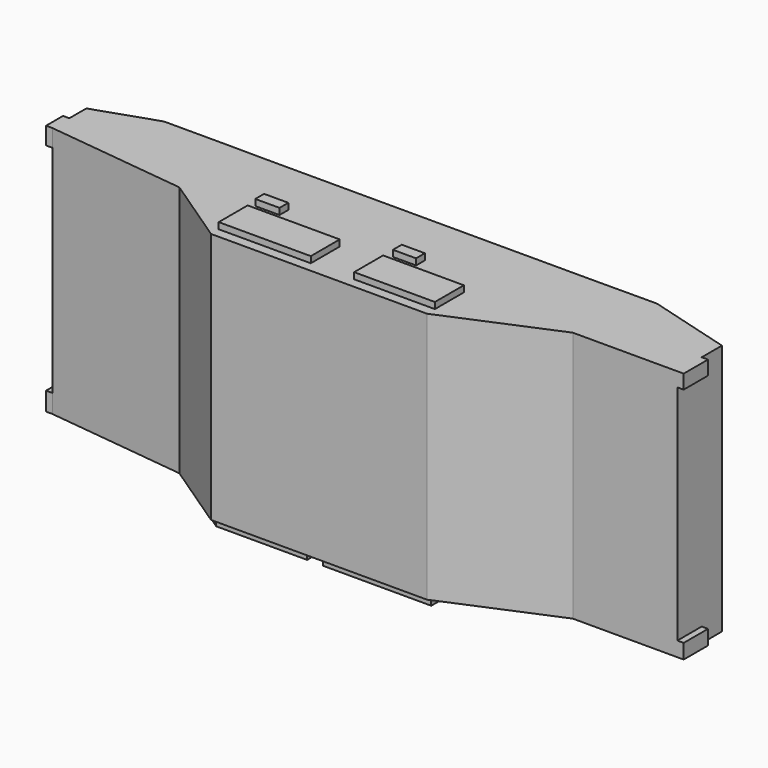
from build123d import *

# Parameters (mm, degrees)
F5_DEPTH  = 127
F6_W      = 54.5970508829
F6_H      = 20.5464081178
F7_DEPTH  = 3.81
F8_W      = 15.3487510979
F8_H      = 7.4063618667
F8_H_2    = 7.1164776087
F9_DEPTH  = 3.175
F10_W     = 10.7039126975
F10_H     = 8.7776441574
F10_H_2   = 9.3331737444
F11_DEPTH = 3.175
F12_W     = 40.7254230231
F12_H     = 18.2523988187
F12_W_2   = 46.4485138655
F13_DEPTH = 3.175
F14_W     = 15.8928539604
F14_H     = 6.1111226678
F14_W_2   = 13.3333727717
F14_H_2   = 5.5555664003
F15_DEPTH = 3.175
F16_W     = 11.666694656
F16_H     = 5.5555701256
F16_W_2   = 12.222263962
F17_DEPTH = 3.175


# Not quite as in the source:
# - the program builds the solid bodies; features that only make, move or delete a surface that nothing else refers to are left out


with BuildPart() as f5:
    # F0 (on Top) → F5 (new body)
    with BuildSketch(Plane.XY):
        with BuildLine():
            Line((94.2318475405, -7.3630477542), (-68.6407278484, -7.3630477542))
            ThreePointArc((-68.6407278484, -7.3630477542), (-68.7653713247, -7.3626377944), (-68.8900094076, -7.3614079328))
            Line((-68.8900094076, -7.3614079328), (-88.84768188, -7.2301225737))
            Line((-88.84768188, -7.2301225737), (-120.7322572041, -7.2301225737))
            Line((-120.7322572041, -7.2301225737), (-151.5727639198, -17.6438004827))
            Line((-151.5727639198, -17.6438004827), (-151.5727639198, -39.0516258776))
            Line((-151.5727639198, -39.0516258776), (-80.8923020959, -47.3129786551))
            Line((-80.8923020959, -47.3129786551), (-46.3170148432, -70.5671533942))
            Line((-46.3170148432, -70.5671533942), (62.6104325056, -70.5671533942))
            Line((62.6104325056, -70.5671533942), (117.5853461027, -47.3129786551))
            Line((117.5853461027, -47.3129786551), (170.3427284956, -47.3129786551))
            Line((170.3427284956, -47.3129786551), (170.3427284956, -19.2245114595))
            Line((170.3427284956, -19.2245114595), (127.9769688845, -7.2301225737))
            Line((127.9769688845, -7.2301225737), (94.2318475405, -7.3630477542))
        make_face()
    extrude(amount=F5_DEPTH)

    # F6 (on face) → F7 (join)
    with BuildSketch(Plane(origin=(0, 0, 0), x_dir=(1, 0, 0), z_dir=(0, 0, -1))):
        Polygon((-45.8669510931, 67.8593867729), (-76.4162167907, 47.3129786551), (0, 47.3129786551), (0, 67.8593867729), align=None)
        with Locations((35.3119070642, 57.586182714)):
            Rectangle(F6_W, F6_H)
    extrude(amount=F7_DEPTH)

    # F8 (on face) → F9 (join)
    with BuildSketch(Plane.YZ.offset(170.3427284956)):
        with Locations((-39.6386031061, 3.7031809334)):
            Rectangle(F8_W, F8_H)
        with Locations((-39.6386031061, 123.4417611957)):
            Rectangle(F8_W, F8_H_2)
    extrude(amount=F9_DEPTH)

    # F10 (on face) → F11 (join)
    with BuildSketch(Plane(origin=(-151.5727639198, 0, 0), x_dir=(0, -1, 0), z_dir=(-1, 0, 0))):
        with Locations((33.6996695289, 122.6111779213)):
            Rectangle(F10_W, F10_H)
        with Locations((33.6996695289, 4.6665868722)):
            Rectangle(F10_W, F10_H_2)
    extrude(amount=F11_DEPTH)

    # F12 (on face) → F13 (join)
    with BuildSketch(Plane.XY.offset(127)):
        with Locations((42.2477209941, -56.4391780645)):
            Rectangle(F12_W, F12_H)
        with Locations((-23.2242569327, -56.4391780645)):
            Rectangle(F12_W_2, F12_H)
    extrude(amount=F13_DEPTH)

    # F14 (on face) → F15 (join)
    with BuildSketch(Plane(origin=(0, 0, 0), x_dir=(1, 0, 0), z_dir=(0, 0, -1))):
        with Locations((-7.9464269802, 38.065303117)):
            Rectangle(F14_W, F14_H)
        with Locations((56.3295595348, 37.7875249833)):
            Rectangle(F14_W_2, F14_H_2)
    extrude(amount=F15_DEPTH)

    # F16 (on face) → F17 (join)
    with BuildSketch(Plane.XY.offset(127)):
        with Locations((27.7183568105, -38.3430793881)):
            Rectangle(F16_W, F16_H)
        with Locations((-41.4484944195, -38.3430793881)):
            Rectangle(F16_W_2, F16_H)
    extrude(amount=F17_DEPTH)


solid = f5.part
